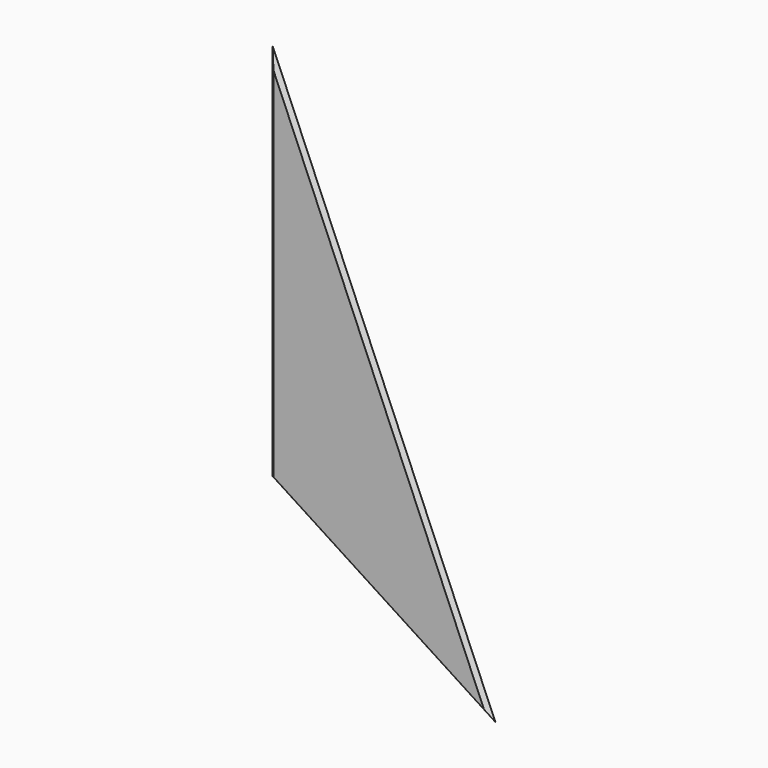
from build123d import *

# Parameters (mm, degrees)
F1_DEPTH = 2.54
F2_SIZE  = 1.26999


# Not quite as in the source:
# - a fillet or chamfer is up to 0.001 mm smaller than in the source, because OpenCascade refuses the exact size


with BuildPart() as f1:
    # F0 (on Front) → F1 (new body)
    with BuildSketch(Plane.XZ):
        Polygon((20.5051476899, -109.5806663148), (-54.1552996701, 65.6793336852), (-54.1552996701, -61.3206663148), align=None)
    extrude(amount=F1_DEPTH)

    # F2 (size 1.27 in the source; OpenCascade refuses exactly that, so slightly less here)
    f2_edges = [f1.edges().sort_by_distance(p)[0] for p in [
        (-16.825076, -2.54, -85.450666),
        (-16.825076, -2.54, -21.950666),
        (-54.1553, -2.54, 2.179334),
        (-16.825076, 0, -85.450666),
        (-16.825076, 0, -21.950666),
        (-54.1553, 0, 2.179334),
    ]]
    chamfer(f2_edges, length=F2_SIZE)


solid = f1.part
